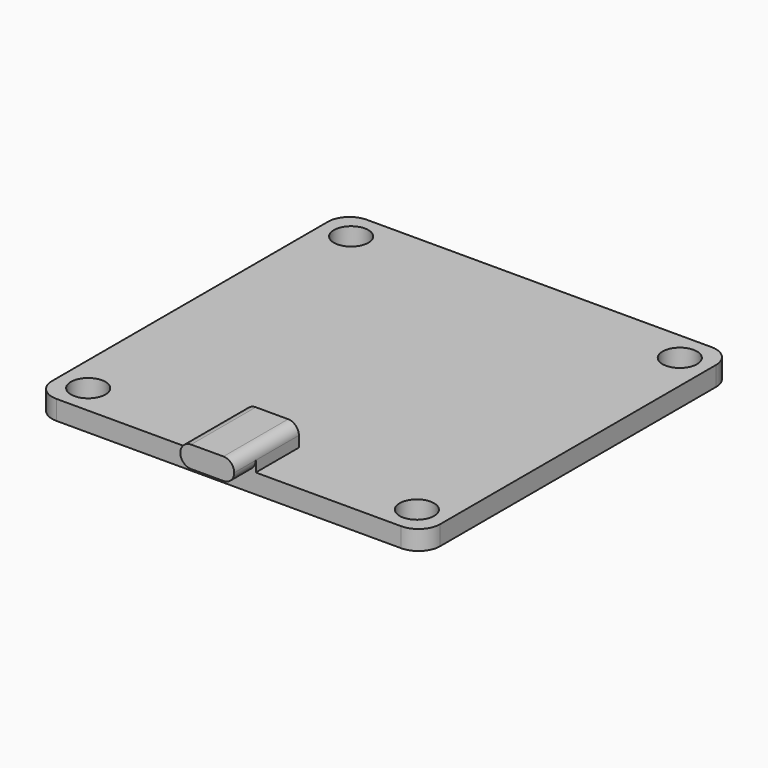
from build123d import *

# Parameters (mm, degrees)
F0_W     = 36
F0_H     = 36
F0_R     = 1.6
F1_DEPTH = 1.8
F2_R     = 2
F3_W     = 5
F3_H     = 7.5
F4_DEPTH = 2
F5_R     = 0.99999


# Not quite as in the source:
# - a fillet or chamfer is up to 0.001 mm smaller than in the source, because OpenCascade refuses the exact size


with BuildPart() as f1:
    # F0 (on Top) → F1 (new body)
    with BuildSketch(Plane.XY):
        Rectangle(F0_W, F0_H)
        with Locations((-15.25, -15.25)):
            Circle(F0_R, mode=Mode.SUBTRACT)
        with Locations((15.25, -15.25)):
            Circle(F0_R, mode=Mode.SUBTRACT)
        with Locations((-15.25, 15.25)):
            Circle(F0_R, mode=Mode.SUBTRACT)
        with Locations((15.25, 15.25)):
            Circle(F0_R, mode=Mode.SUBTRACT)
    extrude(amount=F1_DEPTH)

    # F2
    f2_edges = [f1.edges().sort_by_distance(p)[0] for p in [
        (-18, -18, 0.9),
        (18, -18, 0.9),
        (18, 18, 0.9),
        (-18, 18, 0.9),
    ]]
    fillet(f2_edges, radius=F2_R)

    # F3 (on face) → F4 (join)
    with BuildSketch(Plane.XY.offset(1.8)):
        with Locations((0, -16.75)):
            Rectangle(F3_W, F3_H)
    extrude(amount=F4_DEPTH)

    # F5 (radius 1 in the source; OpenCascade refuses exactly that, so slightly less here)
    f5_edges = [f1.edges().sort_by_distance(p)[0] for p in [
        (-2.5, -19.25, 1.8),
        (-2.5, -16.75, 3.8),
        (2.5, -16.75, 3.8),
        (2.5, -19.25, 1.8),
    ]]
    fillet(f5_edges, radius=F5_R)


solid = f1.part
